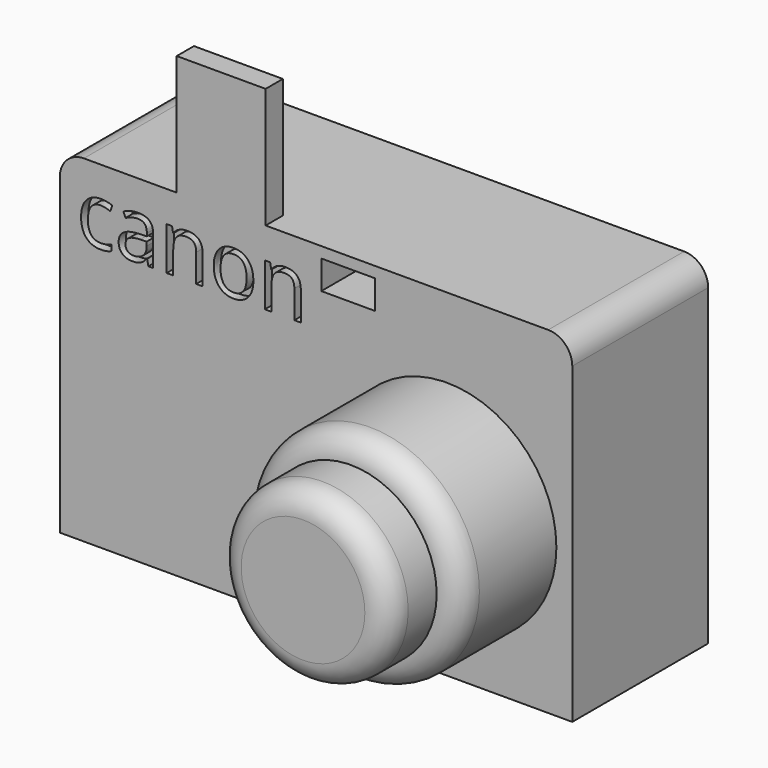
from build123d import *

# Parameters (mm, degrees)
F0_W          = 106.502700597
F0_H          = 35.3089123964
F1_DEPTH      = 70.1
F2_R          = 22.7344676685
F3_DEPTH      = 25
F4_R          = 17.4904081302
F5_DEPTH      = 9.4
F6_R          = 17.8492700396
F7_DEPTH      = 12.4
F8_T1_DEPTH   = 60.3089123964
F9_R          = 6.6746497229
F10_DEPTH     = 4
F11_TEXT_SIZE = 16.748594741
F12_DEPTH     = 1.9
F13_W         = 11.1966878176
F13_H         = 5.9715621173
F14_DEPTH     = 57.4
F16_W         = 18.4745267034
F16_H         = 4.4745588675
F17_DEPTH     = 25


# Not quite as in the source:
# - a fillet or chamfer that OpenCascade refuses, or shapes differently, is made with other operations: its cross-section is extruded or revolved along the edge and cut away or added
# - Text() gives the source's letters only with a copy of the font that has no kerning and outlines rounded to 1/6400 em; it was checked with that copy


with BuildPart() as f1:
    # F0 (on Top) → F1 (new body)
    with BuildSketch(Plane.XY):
        with Locations((-96.3196214288, 23.1636054814)):
            Rectangle(F0_W, F0_H)
    extrude(amount=F1_DEPTH)

    # F2 (on face) → F3 (join)
    with BuildSketch(Plane.XZ.offset(-5.5091492832)):
        with Locations((-69.1036656499, 30.8697484434)):
            Circle(F2_R)
    extrude(amount=F3_DEPTH)

    # F4 (on face) → F5 (join)
    with BuildSketch(Plane.XZ.offset(19.4908507168)):
        with Locations((-69.1036656499, 30.8697484434)):
            Circle(F4_R)
    extrude(amount=-F5_DEPTH)

    # F6 (on face) → F7 (join)
    with BuildSketch(Plane.XZ.offset(19.4908507168)):
        with Locations((-69.1036656499, 30.8697484434)):
            Circle(F6_R)
    extrude(amount=F7_DEPTH)

    # F8: fillet of radius 5 on 4 edges, made by hand

    # F8_s2 → F8_t1 (cut)
    with BuildSketch(Plane.XZ.offset(-53.3180616796)):
        with BuildLine():
            ThreePointArc((-43.0682711303, 65.1), (-44.5327372244, 68.6355339059), (-48.0682711303, 70.1))
            Line((-48.0682711303, 70.1), (-48.0682711303, 70.2))
            Line((-48.0682711303, 70.2), (-42.9682711303, 70.2))
            Line((-42.9682711303, 70.2), (-42.9682711303, 65.1))
            Line((-42.9682711303, 65.1), (-43.0682711303, 65.1))
        make_face()
        with BuildLine():
            ThreePointArc((-149.5709717274, 65.1), (-148.1065056333, 68.6355339059), (-144.5709717274, 70.1))
            Line((-144.5709717274, 70.1), (-144.5709717274, 70.2))
            Line((-144.5709717274, 70.2), (-149.6709717274, 70.2))
            Line((-149.6709717274, 70.2), (-149.6709717274, 65.1))
            Line((-149.6709717274, 65.1), (-149.5709717274, 65.1))
        make_face()
    extrude(amount=F8_T1_DEPTH, mode=Mode.SUBTRACT)

    # F8_s3 → F8_t4 (revolve, cut)
    with BuildSketch(Plane.XY.offset(30.8697484434)):
        with BuildLine():
            ThreePointArc((-51.2543956103, -26.8908507168), (-52.7188617044, -30.4263846228), (-56.2543956103, -31.8908507168))
            Line((-56.2543956103, -31.8908507168), (-56.2543956103, -31.9908507168))
            Line((-56.2543956103, -31.9908507168), (-51.1543956103, -31.9908507168))
            Line((-51.1543956103, -31.9908507168), (-51.1543956103, -26.8908507168))
            Line((-51.1543956103, -26.8908507168), (-51.2543956103, -26.8908507168))
        make_face()
    revolve(axis=Axis((-69.1036656499, -31.8908507168, 30.8697484434), (0, -1, 0)), mode=Mode.SUBTRACT)

    # F8_s5 → F8_t6 (revolve, cut)
    with BuildSketch(Plane.XY.offset(30.8697484434)):
        with BuildLine():
            ThreePointArc((-46.3691979814, -14.492168849), (-47.7933056553, -17.9868782894), (-51.2543956103, -19.4908507168))
            Line((-51.2543956103, -19.4908507168), (-51.2520995629, -19.5908243542))
            ThreePointArc((-51.2520995629, -19.5908243542), (-48.8117967958, -19.5908507168), (-46.3691979814, -19.5908507168))
            Line((-46.3691979814, -19.5908507168), (-46.2691979814, -19.4908507168))
            Line((-46.2691979814, -19.4908507168), (-46.2691979814, -14.492168849))
            Line((-46.2691979814, -14.492168849), (-46.3691979814, -14.492168849))
        make_face()
    revolve(axis=Axis((-69.1036656499, -19.4908507168, 30.8697484434), (0, -1, 0)), mode=Mode.SUBTRACT)

    # F9 (on face) → F10 (join)
    with BuildSketch(Plane.XY.offset(70.1)):
        with Locations((-130.1777362823, 24.706851691)):
            Circle(F9_R)
    extrude(amount=F10_DEPTH)

    # F11 (on face) → F12 (cut)
    with BuildSketch(Plane.XZ.offset(-5.5091492832)):
        with Locations((-146.0859999061, 54.711769335)):
            Text('canon', F11_TEXT_SIZE, font='Open Sans', text_align=(TextAlign.LEFT, TextAlign.BOTTOM))
    extrude(amount=-F12_DEPTH, mode=Mode.SUBTRACT)

    # F13 (on face) → F14 (cut)
    with BuildSketch(Plane.XZ.offset(-5.5091492832)):
        with Locations((-89.6299779415, 64.8474562913)):
            Rectangle(F13_W, F13_H)
    extrude(amount=-F14_DEPTH, mode=Mode.SUBTRACT)

    # F16 (on face) → F17 (join)
    with BuildSketch(Plane.XY.offset(70.1)):
        with Locations((-116.0354875028, 7.7464287169)):
            Rectangle(F16_W, F16_H)
    extrude(amount=F17_DEPTH)


solid = f1.part
